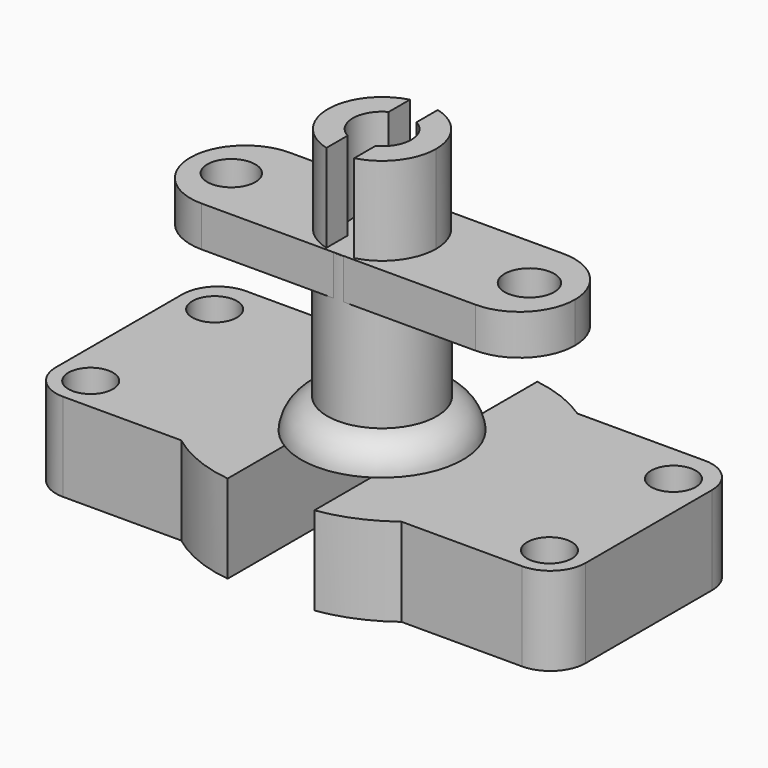
from build123d import *

# Parameters (mm, degrees)
F0_R         = 6.3177385631
F1_DEPTH     = 25
F2_R         = 10
F2_2_R       = 10
F6_DEPTH     = 25
F7_W         = 31.2184179202
F7_H         = 11.4679858088
F8_DEPTH     = 54.5
F9_T1_DEPTH  = 89.929926586
F10_T1_DEPTH = 89.9179858088
F11_R        = 6.8058684083
F11_R_2      = 7.0192014004
F12_DEPTH    = 14.5


# Not quite as in the source:
# - a fillet or chamfer that OpenCascade refuses, or shapes differently, is made with other operations: its cross-section is extruded or revolved along the edge and cut away or added


with BuildPart() as f1:
    # F0 (on Top) → F1 (new body)
    with BuildSketch(Plane.XY):
        with BuildLine():
            Line((-29.585074326, 33.0942198634), (-75.0644803047, 33.0942198634))
            Line((-75.0644803047, 33.0942198634), (-75.0644803047, -31.6854342818))
            Line((-75.0644803047, -31.6854342818), (-31.5542415078, -31.6854342818))
            ThreePointArc((-31.5542415078, -31.6854342818), (-47.222641265, 1.2106089588), (-29.585074326, 33.0942198634))
        make_face()
        with Locations((-64.9971365929, -21.9507273287)):
            Circle(F0_R, mode=Mode.SUBTRACT)
        with Locations((-64.9971365929, 21.9507273287)):
            Circle(F0_R, mode=Mode.SUBTRACT)
        with BuildLine():
            ThreePointArc((-12.1024890528, 39.5649749036), (-21.2275389144, 37.3664266823), (-29.585074326, 33.0942198634))
            Line((-29.585074326, 33.0942198634), (-12.1024890528, 33.0942198634))
            Line((-12.1024890528, 33.0942198634), (-12.1024890528, 39.5649749036))
        make_face()
        with BuildLine():
            Line((-12.1024890528, 33.0942198634), (-29.585074326, 33.0942198634))
            ThreePointArc((-29.585074326, 33.0942198634), (-47.222641265, 1.2106089588), (-31.5542415078, -31.6854342818))
            Line((-31.5542415078, -31.6854342818), (-12.1024890528, -31.6854342818))
            Line((-12.1024890528, -31.6854342818), (-12.1024890528, 33.0942198634))
        make_face()
        with BuildLine():
            Line((-12.1024890528, -31.6854342818), (-31.5542415078, -31.6854342818))
            ThreePointArc((-31.5542415078, -31.6854342818), (-22.3564909939, -36.9289570753), (-12.1024890528, -39.5649749036))
            Line((-12.1024890528, -39.5649749036), (-12.1024890528, -31.6854342818))
        make_face()
    extrude(amount=F1_DEPTH)

    # F2
    f2_edges = [f1.edges().sort_by_distance(p)[0] for p in [
        (-75.06448, 33.09422, 12.5),
        (-75.06448, -31.685434, 12.5),
    ]]
    fillet(f2_edges, radius=F2_R)


with BuildPart() as f1b:
    # F0 (on Top) → F1, piece 2 (new body)
    with BuildSketch(Plane.XY):
        with BuildLine():
            Line((75.027666986, 22.9723975062), (75.027666986, 33.0942198634))
            Line((75.027666986, 33.0942198634), (28.8700831713, 33.0942198634))
            ThreePointArc((28.8700831713, 33.0942198634), (46.4635935741, 1.2073128731), (30.8311391826, -31.6854342818))
            Line((30.8311391826, -31.6854342818), (75.027666986, -31.6854342818))
            Line((75.027666986, -31.6854342818), (75.027666986, -23.3383905143))
            Line((75.027666986, -23.3383905143), (75.027666986, 22.9723975062))
        make_face()
        with Locations((64.9971365929, -21.9507273287)):
            Circle(F0_R, mode=Mode.SUBTRACT)
        with Locations((64.9971365929, 21.9507273287)):
            Circle(F0_R, mode=Mode.SUBTRACT)
        with BuildLine():
            ThreePointArc((30.8311391826, -31.6854342818), (46.4635935741, 1.2073128731), (28.8700831713, 33.0942198634))
            Line((28.8700831713, 33.0942198634), (12.3979339147, 33.0942198634))
            Line((12.3979339147, 33.0942198634), (12.3979339147, -31.6854342818))
            Line((12.3979339147, -31.6854342818), (30.8311391826, -31.6854342818))
        make_face()
        with BuildLine():
            Line((12.3979339147, 33.0942198634), (28.8700831713, 33.0942198634))
            ThreePointArc((28.8700831713, 33.0942198634), (20.991464616, 37.2068208279), (12.3979339147, 39.4733924947))
            Line((12.3979339147, 39.4733924947), (12.3979339147, 33.0942198634))
        make_face()
        with BuildLine():
            ThreePointArc((12.3979339147, -39.4733924947), (22.1107023598, -36.7537810458), (30.8311391826, -31.6854342818))
            Line((30.8311391826, -31.6854342818), (12.3979339147, -31.6854342818))
            Line((12.3979339147, -31.6854342818), (12.3979339147, -39.4733924947))
        make_face()
    extrude(amount=F1_DEPTH)

    # F2#2
    f2_2_edges = [f1b.edges().sort_by_distance(p)[0] for p in [
        (75.027667, 33.09422, 12.5),
        (75.027667, -31.685434, 12.5),
    ]]
    fillet(f2_2_edges, radius=F2_2_R)


with BuildPart() as f4:
    # F3 (on Right) → F4 (revolve)
    with BuildSketch(Plane.YZ):
        with BuildLine():
            Line((-15.5135737732, 24.9761715531), (-15.5135737732, 33.4417130729))
            ThreePointArc((-15.5135737732, 33.4417130729), (-20.5636997877, 30.386116132), (-22.924408385, 24.9761715531))
            Line((-22.924408385, 24.9761715531), (-15.5135737732, 24.9761715531))
        make_face()
        Polygon((0, 24.9761715531), (0, 75.0537067652), (-15.5135737732, 75.0537067652), (-15.5135737732, 33.4417130729), (-15.5135737732, 24.9761715531), align=None)
    revolve(axis=Axis((0, 0, 50.0149391592), (0, 0, -1)))

    # F5 (on face) → F6 (join)
    with BuildSketch(Plane.XY.offset(75.0537067652)):
        with BuildLine():
            ThreePointArc((-3.94382999, -7.2839486676), (-8.2830974389, 0), (-3.94382999, 7.2839486676))
            Line((-3.94382999, 7.2839486676), (-3.94382999, 14.7966654673))
            ThreePointArc((-3.94382999, 14.7966654673), (-15.3132329683, 0), (-3.94382999, -14.7966654673))
            Line((-3.94382999, -14.7966654673), (-3.94382999, -7.2839486676))
        make_face()
        with BuildLine():
            ThreePointArc((3.94382999, 7.2839486676), (7.1160674277, 4.2392555415), (8.2830974389, 0))
            ThreePointArc((8.2830974389, 0), (7.1160674277, -4.2392555415), (3.94382999, -7.2839486676))
            Line((3.94382999, -7.2839486676), (3.94382999, -14.7966654673))
            ThreePointArc((3.94382999, -14.7966654673), (12.1426498625, -9.3301210206), (15.3132329683, 0))
            ThreePointArc((15.3132329683, 0), (12.1426498625, 9.3301210206), (3.94382999, 14.7966654673))
            Line((3.94382999, 14.7966654673), (3.94382999, 7.2839486676))
        make_face()
    extrude(amount=F6_DEPTH)

    # F7 (on Right) → F8 (join, symmetric)
    with BuildSketch(Plane.YZ):
        with Locations((0.1592780463, 69.3889670074)):
            Rectangle(F7_W, F7_H)
    extrude(amount=F8_DEPTH, both=True)

    # F9: fillet of radius 15.6923881554 on 2 edges, made by hand

    # F9_s2 → F9_t1 (cut)
    with BuildSketch(Plane.XY.offset(24.4240037144)):
        with BuildLine():
            ThreePointArc((38.8076118446, -15.4499309137), (49.9038059223, -10.853736836), (54.5, 0.2424572417))
            Line((54.5, 0.2424572417), (54.5, -15.4499309137))
            Line((54.5, -15.4499309137), (38.8076118446, -15.4499309137))
        make_face()
        with BuildLine():
            ThreePointArc((54.5, 0.076098851), (49.9038059223, 11.1722929287), (38.8076118446, 15.7684870064))
            Line((38.8076118446, 15.7684870064), (54.5, 15.7684870064))
            Line((54.5, 15.7684870064), (54.5, 0.076098851))
        make_face()
    extrude(amount=F9_T1_DEPTH, mode=Mode.SUBTRACT)

    # F10: fillet of radius 15.69 on 2 edges, made by hand

    # F10_s2 → F10_t1 (cut)
    with BuildSketch(Plane.XY.offset(24.429974103)):
        with BuildLine():
            ThreePointArc((-38.81, -15.4499309137), (-49.9045053968, -10.8544363106), (-54.5, 0.2400690863))
            Line((-54.5, 0.2400690863), (-54.5, -15.4499309137))
            Line((-54.5, -15.4499309137), (-38.81, -15.4499309137))
        make_face()
        with BuildLine():
            ThreePointArc((-54.5, 0.0784870064), (-49.9045053968, 11.1729924032), (-38.81, 15.7684870064))
            Line((-38.81, 15.7684870064), (-54.5, 15.7684870064))
            Line((-54.5, 15.7684870064), (-54.5, 0.0784870064))
        make_face()
    extrude(amount=F10_T1_DEPTH, mode=Mode.SUBTRACT)

    # F11 (on face) → F12 (cut)
    with BuildSketch(Plane.XY.offset(75.1229599118)):
        with Locations((-42.7188128233, 0)):
            Circle(F11_R)
        with Locations((41.626945138, 0.1592780463)):
            Circle(F11_R_2)
    extrude(amount=-F12_DEPTH, mode=Mode.SUBTRACT)


solid = Compound([f1.part, f1b.part, f4.part])
